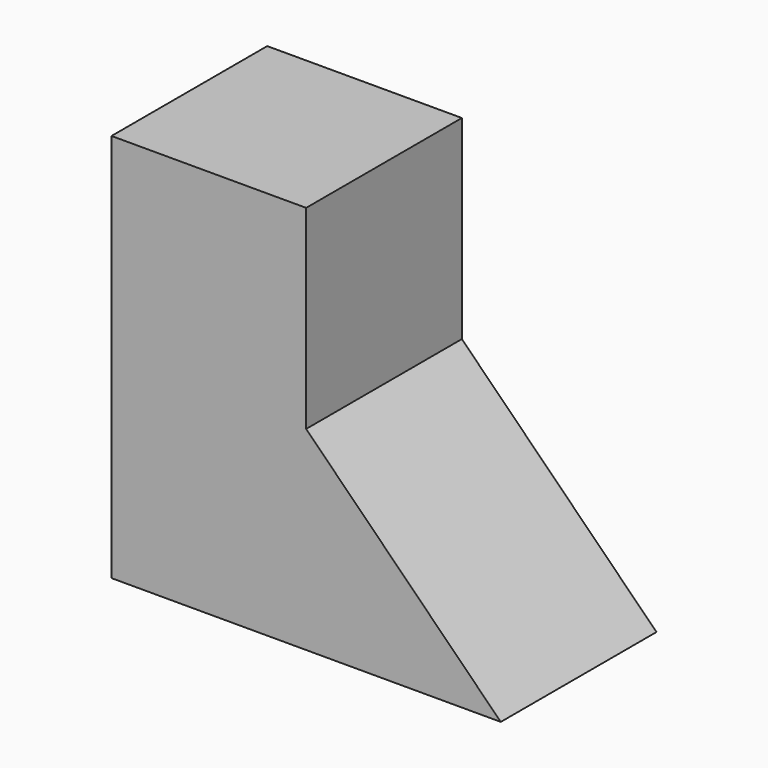
from build123d import *

# Parameters (mm, degrees)
F1_DEPTH = 25


with BuildPart() as f1:
    # F0 (on Front) → F1 (new body)
    with BuildSketch(Plane.XZ):
        Polygon((0, 0), (-25, 25), (-25, -25), (25, -25), align=None)
        Polygon((0, 25), (-25, 25), (0, 0), align=None)
    extrude(amount=-F1_DEPTH)


solid = f1.part
